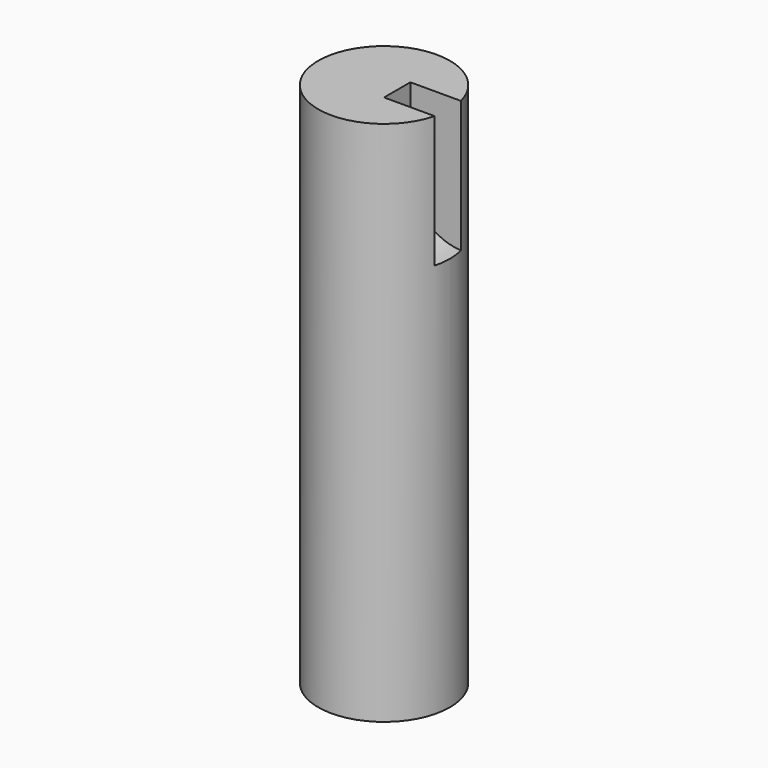
from build123d import *

# Parameters (mm, degrees)
F0_R     = 3.175
F1_DEPTH = 25.4
F2_W     = 2.54
F2_H     = 1.5875
F3_DEPTH = 6.35
F4_R     = 2.53999


# Not quite as in the source:
# - a fillet or chamfer is up to 0.001 mm smaller than in the source, because OpenCascade refuses the exact size


with BuildPart() as f1:
    # F0 (on Top) → F1 (new body)
    with BuildSketch(Plane.XY):
        Circle(F0_R)
    extrude(amount=F1_DEPTH)

    # F2 (on face) → F3 (cut)
    with BuildSketch(Plane.XY.offset(25.4)):
        with Locations((1.905, 0)):
            Rectangle(F2_W, F2_H)
    extrude(amount=-F3_DEPTH, mode=Mode.SUBTRACT)

    # F4 (radius 2.54 in the source; OpenCascade refuses exactly that, so slightly less here)
    f4_edges = [f1.edges().sort_by_distance(p)[0] for p in [
        (0.635, 0, 19.05),
    ]]
    fillet(f4_edges, radius=F4_R)


solid = f1.part
